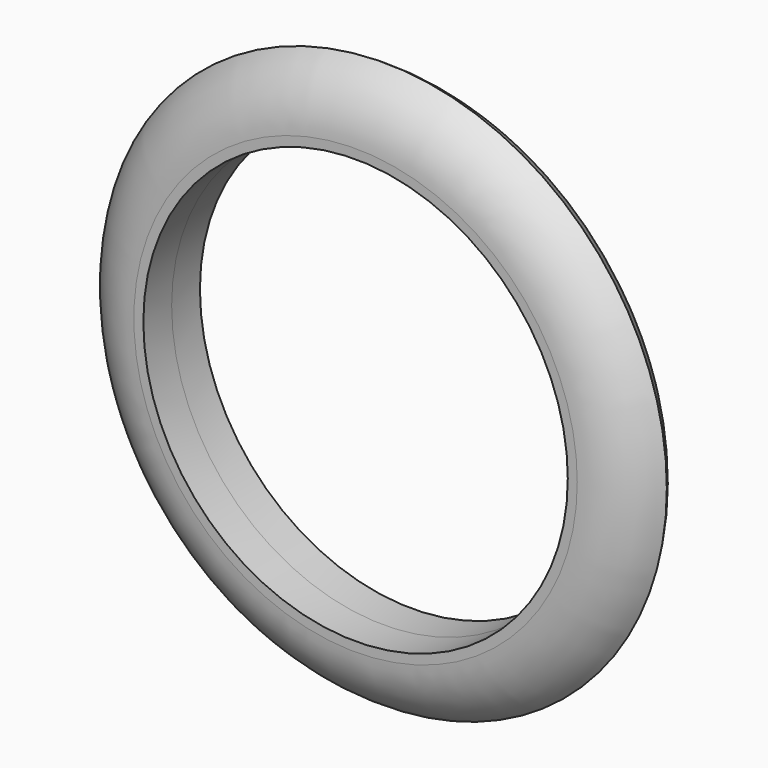
from build123d import *

# Parameters (mm, degrees)
F0_R     = 20
F0_R_2   = 15
F1_DEPTH = 2.5


# Not quite as in the source:
# - a fillet or chamfer that OpenCascade refuses, or shapes differently, is made with other operations: its cross-section is extruded or revolved along the edge and cut away or added


with BuildPart() as f1:
    # F0 (on Front) → F1 (new body)
    with BuildSketch(Plane.XZ):
        Circle(F0_R)
        Circle(F0_R_2, mode=Mode.SUBTRACT)
    extrude(amount=F1_DEPTH)

    # F2: fillet of radius 5 on 1 edges, made by hand

    # F2_s1 → F2_t2 (revolve, cut)
    with BuildSketch(Plane.XY):
        with BuildLine():
            ThreePointArc((20, 0), (18.1698729811, -1.8301270189), (15.6698729811, -2.5))
            Line((15.6698729811, -2.5), (20, -2.5))
            Line((20, -2.5), (20, 0))
        make_face()
    revolve(axis=Axis((0, -2.5, 0), (0, -1, 0)), mode=Mode.SUBTRACT)

    # F3: F1 across plane


with BuildPart() as f1_1:
    add(f1.part)
    add(f1.part.mirror(Plane.XZ))


solid = f1_1.part
